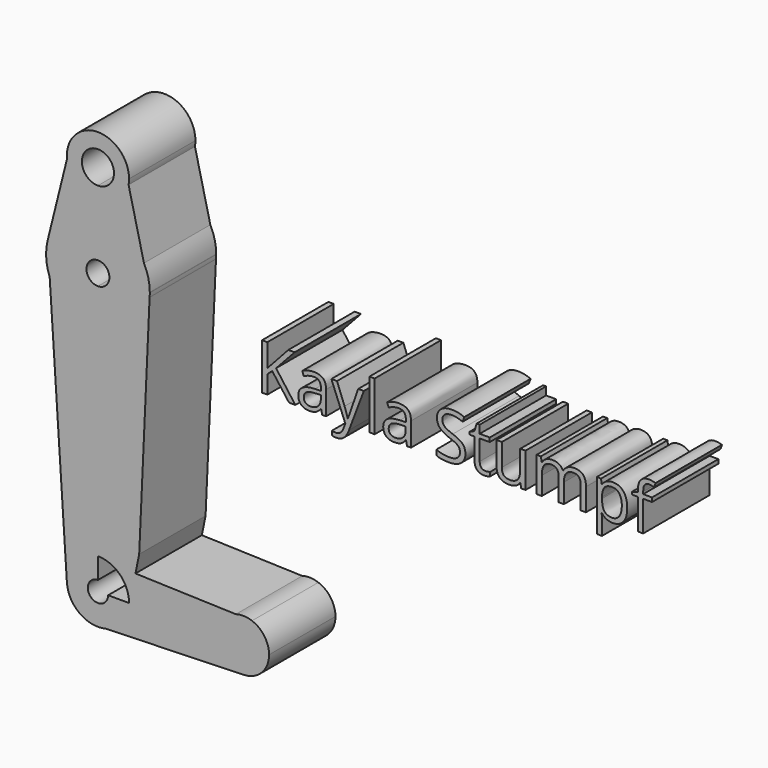
from build123d import *

# Parameters (mm, degrees)
F0_TEXT_SIZE = 19.7987796532
F1_DEPTH     = 25.4


# Not quite as in the source:
# - Text() gives the source's letters only with a copy of the font that has no kerning and outlines rounded to 1/6400 em; it was checked with that copy


with BuildPart() as f1:
    # F0 (on Front) → F1 (new body)
    with BuildSketch(Plane.XZ):
        with BuildLine():
            ThreePointArc((-42.0644047008, 51.8182271492), (-39.0017716721, 45.6466855883), (-32.5784642483, 43.1549456247))
            ThreePointArc((-32.5784642483, 43.1549456247), (-26.4557750258, 45.3834874644), (-23.1981081873, 51.0262996016))
            ThreePointArc((-23.1981081873, 51.0262996016), (-23.0896941362, 51.8499656492), (-23.0534642483, 52.6799456247))
            ThreePointArc((-23.0534642483, 52.6799456247), (-33.0097658768, 62.1951757272), (-42.0644047008, 51.8182271492))
        make_face()
        with BuildLine():
            ThreePointArc((-27.6628373258, 52.6799456247), (-29.1025911176, 49.204072494), (-32.5784642483, 47.7643187022))
            ThreePointArc((-32.5784642483, 47.7643187022), (-36.0543373789, 56.1558187553), (-27.6628373258, 52.6799456247))
        make_face(mode=Mode.SUBTRACT)
        with BuildLine():
            ThreePointArc((-23.1981081873, 51.0262996016), (-26.4557750258, 45.3834874644), (-32.5784642483, 43.1549456247))
            Line((-32.5784642483, 43.1549456247), (-32.5784642483, 40.0274897093))
            ThreePointArc((-32.5784642483, 40.0274897093), (-24.3355255959, 37.7197144577), (-18.4891664487, 31.4673589847))
            Line((-18.4891664487, 31.4673589847), (-23.1981081873, 51.0262996016))
        make_face()
        with BuildLine():
            Line((-32.5784642483, 40.0274897093), (-32.5784642483, 43.1549456247))
            ThreePointArc((-32.5784642483, 43.1549456247), (-39.0017716721, 45.6466855883), (-42.0644047008, 51.8182271492))
            Line((-42.0644047008, 51.8182271492), (-47.9853613834, 27.9791260477))
            ThreePointArc((-47.9853613834, 27.9791260477), (-42.3577222244, 36.6577581365), (-32.5784642483, 40.0274897093))
        make_face()
        with BuildLine():
            ThreePointArc((-18.4891664487, 31.4673589847), (-24.3355255959, 37.7197144577), (-32.5784642483, 40.0274897093))
            Line((-32.5784642483, 40.0274897093), (-32.5784642483, 27.6581364439))
            ThreePointArc((-32.5784642483, 27.6581364439), (-30.0995976698, 26.6313562877), (-29.0728175137, 24.1524897093))
            ThreePointArc((-29.0728175137, 24.1524897093), (-30.0995976698, 21.6736231308), (-32.5784642483, 20.6468429747))
            Line((-32.5784642483, 20.6468429747), (-32.5784642483, 8.2774897093))
            ThreePointArc((-32.5784642483, 8.2774897093), (-21.8367280075, 12.4635749806), (-16.7599774507, 22.814169705))
            Line((-16.7599774507, 22.814169705), (-16.7037845731, 24.0516422435))
            Line((-16.7037845731, 24.0516422435), (-18.4891664487, 31.4673589847))
        make_face()
        with BuildLine():
            Line((-32.5784642483, 27.6581364439), (-32.5784642483, 40.0274897093))
            ThreePointArc((-32.5784642483, 40.0274897093), (-42.3577222244, 36.6577581365), (-47.9853613834, 27.9791260477))
            Line((-47.9853613834, 27.9791260477), (-47.3555091533, 18.3512339077))
            ThreePointArc((-47.3555091533, 18.3512339077), (-41.5205190778, 11.0355052835), (-32.5784642483, 8.2774897093))
            Line((-32.5784642483, 8.2774897093), (-32.5784642483, 20.6468429747))
            ThreePointArc((-32.5784642483, 20.6468429747), (-36.0841109829, 24.1524897093), (-32.5784642483, 27.6581364439))
        make_face()
        with BuildLine():
            ThreePointArc((-16.7034642483, 24.1524897093), (-17.1563498088, 27.9173285128), (-18.4891664487, 31.4673589847))
            Line((-18.4891664487, 31.4673589847), (-16.7037845731, 24.0516422435))
            ThreePointArc((-16.7037845731, 24.0516422435), (-16.7035443297, 24.102065722), (-16.7034642483, 24.1524897093))
        make_face()
        with BuildLine():
            Line((-47.3555091533, 18.3512339077), (-47.9853613834, 27.9791260477))
            ThreePointArc((-47.9853613834, 27.9791260477), (-48.4196026555, 23.1161697954), (-47.3555091533, 18.3512339077))
        make_face()
        with BuildLine():
            ThreePointArc((-16.7599774507, 22.814169705), (-16.719806208, 23.4323576647), (-16.7037845731, 24.0516422435))
            Line((-16.7037845731, 24.0516422435), (-16.7599774507, 22.814169705))
        make_face()
        with BuildLine():
            ThreePointArc((-32.5784642483, 8.2774897093), (-41.5205190778, 11.0355052835), (-47.3555091533, 18.3512339077))
            Line((-47.3555091533, 18.3512339077), (-42.0831472926, -62.2418463237))
            ThreePointArc((-42.0831472926, -62.2418463237), (-39.5300177908, -55.108408781), (-32.5784642483, -52.0950543753))
            Line((-32.5784642483, -52.0950543753), (-32.5784642483, 8.2774897093))
        make_face()
        with BuildLine():
            ThreePointArc((-16.7599774507, 22.814169705), (-21.8367280075, 12.4635749806), (-32.5784642483, 8.2774897093))
            Line((-32.5784642483, 8.2774897093), (-32.5784642483, -52.0950543753))
            ThreePointArc((-32.5784642483, -52.0950543753), (-30.7842782896, -52.2655623129), (-29.0543281205, -52.7709815678))
            Line((-29.0543281205, -52.7709815678), (-21.092662713, -53.0246133955))
            Line((-21.092662713, -53.0246133955), (-19.9509463802, -47.4569499493))
            Line((-19.9509463802, -47.4569499493), (-16.7599774507, 22.814169705))
        make_face()
        with BuildLine():
            ThreePointArc((-32.5784642483, -52.0950543753), (-39.5300177908, -55.108408781), (-42.0831472926, -62.2418463237))
            ThreePointArc((-42.0831472926, -62.2418463237), (-39.6812731575, -67.9663706769), (-34.2622093374, -70.9950545073))
            Line((-34.2622093374, -70.9950545073), (-30.3143133192, -70.8720404092))
            ThreePointArc((-30.3143133192, -70.8720404092), (-25.0854120464, -67.5005130054), (-23.0534642483, -61.6200543753))
            Line((-23.0534642483, -61.6200543753), (-29.473796058, -61.6200543753))
            ThreePointArc((-29.473796058, -61.6200543753), (-34.7737961789, -63.815386306), (-32.5784642483, -58.5153861851))
            Line((-32.5784642483, -58.5153861851), (-32.5784642483, -52.0950543753))
        make_face()
        with BuildLine():
            Line((-30.3143133192, -70.8720404092), (-34.2622093374, -70.9950545073))
            ThreePointArc((-34.2622093374, -70.9950545073), (-32.281814873, -71.1404337873), (-30.3143133192, -70.8720404092))
        make_face()
        with BuildLine():
            Line((-21.092662713, -53.0246133955), (-29.0543281205, -52.7709815678))
            ThreePointArc((-29.0543281205, -52.7709815678), (-24.6951584183, -56.2741106615), (-23.0534642483, -61.6200543753))
            Line((-23.0534642483, -61.6200543753), (-22.8552612338, -61.6200543753))
            Line((-22.8552612338, -61.6200543753), (-21.092662713, -53.0246133955))
        make_face()
        with BuildLine():
            Line((9.637056071, -54.0035586715), (-21.092662713, -53.0246133955))
            Line((-21.092662713, -53.0246133955), (-22.8552612338, -61.6200543753))
            Line((-22.8552612338, -61.6200543753), (3.9340357517, -61.6200543753))
            ThreePointArc((3.9340357517, -61.6200543753), (5.5177932044, -56.8625485275), (9.637056071, -54.0035586715))
        make_face()
        with BuildLine():
            ThreePointArc((-23.0534642483, -61.6200543753), (-25.0854120464, -67.5005130054), (-30.3143133192, -70.8720404092))
            Line((-30.3143133192, -70.8720404092), (11.8715357517, -69.5575543753))
            ThreePointArc((11.8715357517, -69.5575543753), (6.2588756761, -67.232714451), (3.9340357517, -61.6200543753))
            Line((3.9340357517, -61.6200543753), (-22.8552612338, -61.6200543753))
            Line((-22.8552612338, -61.6200543753), (-23.0534642483, -61.6200543753))
        make_face()
        with BuildLine():
            Line((14.5862645222, -54.1612237731), (9.637056071, -54.0035586715))
            ThreePointArc((9.637056071, -54.0035586715), (5.5177932044, -56.8625485275), (3.9340357517, -61.6200543753))
            ThreePointArc((3.9340357517, -61.6200543753), (6.2588756761, -67.232714451), (11.8715357517, -69.5575543753))
            ThreePointArc((11.8715357517, -69.5575543753), (17.4841958274, -67.232714451), (19.8090357517, -61.6200543753))
            ThreePointArc((19.8090357517, -61.6200543753), (18.3735379766, -57.0672669525), (14.5862645222, -54.1612237731))
        make_face()
        with BuildLine():
            ThreePointArc((14.5862645222, -54.1612237731), (12.1242695407, -53.6865789779), (9.637056071, -54.0035586715))
            Line((9.637056071, -54.0035586715), (14.5862645222, -54.1612237731))
        make_face()
        with Locations((15.6986713409, 8.300408721)):
            Text('Kayla Stumpf', F0_TEXT_SIZE, font='Open Sans', text_align=(TextAlign.LEFT, TextAlign.BOTTOM))
    extrude(amount=F1_DEPTH)


solid = f1.part
